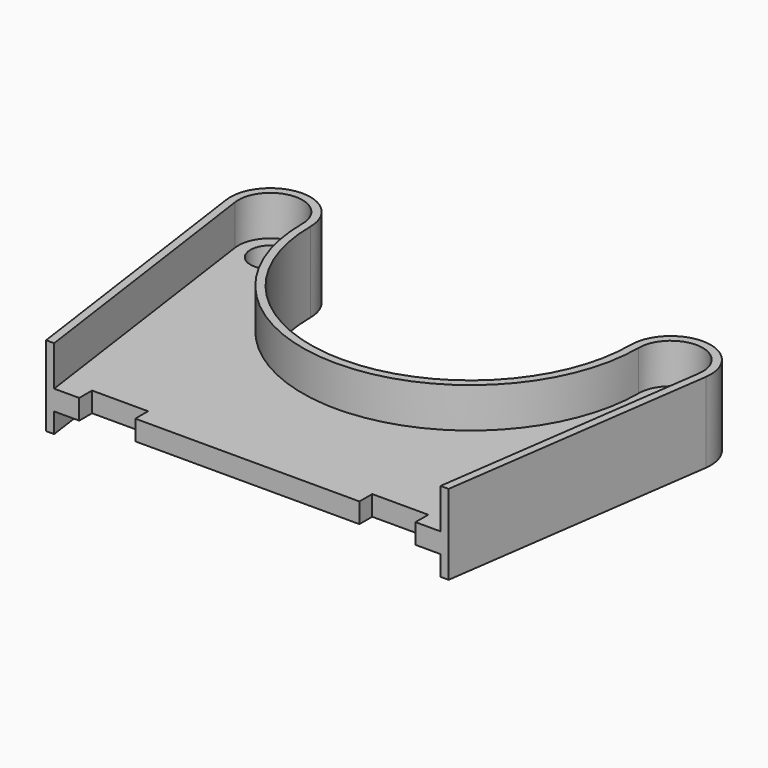
from build123d import *

# Parameters (mm, degrees)
F0_R     = 5
F1_DEPTH = 2.5
F3_DEPTH = 10


# Not quite as in the source:
# - a feature names something its author has since deleted; it is built from what else it names


with BuildPart() as f1:
    # F0 (on Top) → F1 (new body, symmetric)
    with BuildSketch(Plane.XY):
        with BuildLine():
            ThreePointArc((2.8545027599, -6.0492269011), (0, -6.146341392), (-2.8545027599, -6.0492269011))
            ThreePointArc((-2.8545027599, -6.0492269011), (-30.6911152935, 7.182149369), (-42, 35.853658608))
            ThreePointArc((-42, 35.853658608), (-50.5591908622, 43.8340912767), (-57.9218263949, 34.7380123518))
            Line((-57.9218263949, 34.7380123518), (-48.2619276413, -33.853658608))
            Line((-48.2619276413, -33.853658608), (-42, -33.853658608))
            Line((-42, -33.853658608), (-42, -29.853658608))
            Line((-42, -29.853658608), (-28, -29.853658608))
            Line((-28, -29.853658608), (-28, -33.853658608))
            Line((-28, -33.853658608), (28, -33.853658608))
            Line((28, -33.853658608), (28, -29.853658608))
            Line((28, -29.853658608), (42, -29.853658608))
            Line((42, -29.853658608), (42, -33.853658608))
            Line((42, -33.853658608), (48.2619276413, -33.853658608))
            Line((48.2619276413, -33.853658608), (57.9218263949, 34.7380123518))
            ThreePointArc((57.9218263949, 34.7380123518), (50.5591908622, 43.8340912767), (42, 35.853658608))
            ThreePointArc((42, 35.853658608), (30.6911152935, 7.182149369), (2.8545027599, -6.0492269011))
        make_face()
        with Locations((-50, 35.853658608)):
            Circle(F0_R, mode=Mode.SUBTRACT)
        with Locations((50, 35.853658608)):
            Circle(F0_R, mode=Mode.SUBTRACT)
    extrude(amount=F1_DEPTH, both=True)

    # F2 (on face) → F3 (join, symmetric)
    with BuildSketch(Plane.XY.offset(2.5)):
        with BuildLine():
            Line((48.2619276413, -33.853658608), (50.2816638994, -33.853658608))
            Line((50.2816638994, -33.853658608), (59.9022829936, 34.4591007877))
            ThreePointArc((59.9022829936, 34.4591007877), (50.6989885778, 45.8291994439), (40, 35.853658608))
            ThreePointArc((40, 35.853658608), (0, -4.146341392), (-40, 35.853658608))
            ThreePointArc((-40, 35.853658608), (-50.6989885778, 45.8291994439), (-59.9022829936, 34.4591007877))
            Line((-59.9022829936, 34.4591007877), (-50.2816638994, -33.853658608))
            Line((-50.2816638994, -33.853658608), (-48.2619276413, -33.853658608))
            Line((-48.2619276413, -33.853658608), (-57.9218263949, 34.7380123518))
            ThreePointArc((-57.9218263949, 34.7380123518), (-50.5591908622, 43.8340912767), (-42, 35.853658608))
            ThreePointArc((-42, 35.853658608), (0, -6.146341392), (42, 35.853658608))
            ThreePointArc((42, 35.853658608), (50.5591908622, 43.8340912767), (57.9218263949, 34.7380123518))
            Line((57.9218263949, 34.7380123518), (48.2619276413, -33.853658608))
        make_face()
    extrude(amount=F3_DEPTH, both=True)


solid = f1.part
